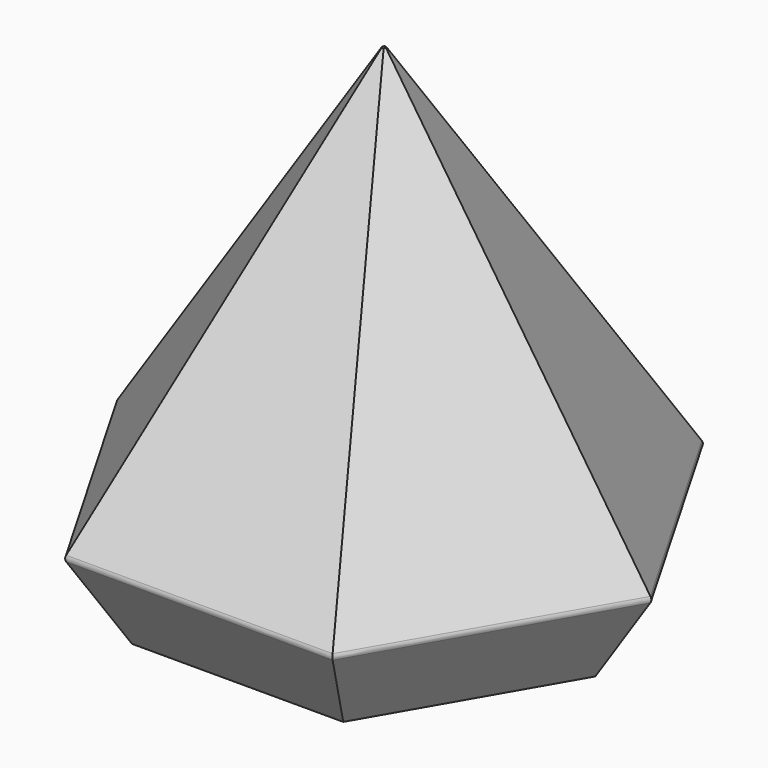
from build123d import *

# Parameters (mm, degrees)
F1_DEPTH = 15
F1_TAPER = -30
F2_DEPTH = 15
F2_TAPER = -30
F3_DEPTH = 1
F3_TAPER = -35
F5_DEPTH = 70
F5_TAPER = 30
F9_R     = 1


# Not quite as in the source:
# - an extrude whose draft closes it to a point is written as a loft to that point


with BuildPart() as f1:
    # F0 (on Top) → F1 (new body)
    with BuildSketch(Plane.XY):
        Polygon((-18.4989116336, 32.043568284), (-36.9999999787, 0.0012567249), (-18.501088345, -32.0423115591), (18.4989116336, -32.043568284), (36.9999999787, -0.0012567249), (18.501088345, 32.0423115591), align=None)
        Polygon((17.57727357, 30.442342936), (35.1524791183, -0.0011939729), (17.5752055483, -30.4435369089), (-17.57727357, -30.442342936), (-35.1524791183, 0.0011939729), (-17.5752055483, 30.4435369089), align=None, mode=Mode.SUBTRACT)
    extrude(amount=F1_DEPTH, taper=F1_TAPER)

    # F0 (on Top) → F2 (cut)
    with BuildSketch(Plane.XY):
        Polygon((17.5752055483, -30.4435369089), (35.1524791183, -0.0011939729), (17.57727357, 30.442342936), (-17.5752055483, 30.4435369089), (-35.1524791183, 0.0011939729), (-17.57727357, -30.442342936), align=None)
    extrude(amount=F2_DEPTH, taper=F2_TAPER, mode=Mode.SUBTRACT)

    # F0 (on Top) → F3 (join)
    with BuildSketch(Plane.XY):
        Polygon((17.5752055483, -30.4435369089), (35.1524791183, -0.0011939729), (17.57727357, 30.442342936), (-17.5752055483, 30.4435369089), (-35.1524791183, 0.0011939729), (-17.57727357, -30.442342936), align=None)
    extrude(amount=F3_DEPTH, taper=F3_TAPER)


with BuildPart() as f5:
    # F4 (on face) → F5 (new body)
    with BuildSketch(Plane.XY.offset(15)):
        Polygon((23.4986174805, -40.7039921445), (46.9999999729, -0.0015963803), (23.5013824923, 40.7023957642), (-23.4986174805, 40.7039921445), (-46.9999999729, 0.0015963803), (-23.5013824923, -40.7023957642), align=None)
    extrude(amount=F5_DEPTH, taper=F5_TAPER)

    # F6 (on face) → F7 section 0
    with BuildSketch(Plane(origin=(0, 0, 15), x_dir=(1, 0, 0), z_dir=(0, 0, -1)), mode=Mode.PRIVATE) as f7_s0:
        Polygon((45.3999999738, 0.0015420354), (22.698664545, 39.3183243269), (-22.7013354288, 39.3167822914), (-45.3999999738, -0.0015420354), (-22.698664545, -39.3183243269), (22.7013354288, -39.3167822914), align=None)
    loft([f7_s0.sketch, Vertex(0, 0, 83.1)], ruled=True, mode=Mode.SUBTRACT)


with BuildPart() as f1_1:
    add(f1.part)

    # F8: union F5
    add(f5.part)

    # F9
    f9_edges = [f1_1.edges().sort_by_distance(p)[0] for p in [
        (-0.001383, -40.703194, 15),
        (35.249309, -20.352794, 15),
        (35.250691, 20.3504, 15),
        (0.001383, 40.703194, 15),
        (-35.249309, 20.352794, 15),
        (-35.250691, -20.3504, 15),
    ]]
    fillet(f9_edges, radius=F9_R)


solid = f1_1.part
